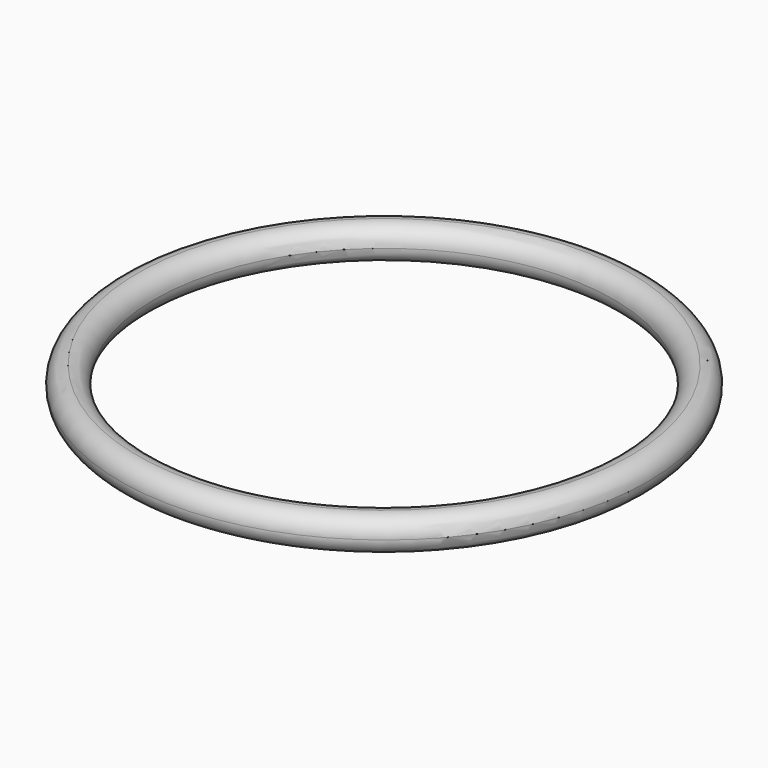
from build123d import *

# Parameters (mm, degrees)
F0_R     = 11.5
F0_R_2   = 10
F1_DEPTH = 1.5
F2_R     = 0.74999


# Not quite as in the source:
# - a fillet or chamfer is up to 0.001 mm smaller than in the source, because OpenCascade refuses the exact size


with BuildPart() as f1:
    # F0 (on Top) → F1 (new body)
    with BuildSketch(Plane.XY):
        Circle(F0_R)
        Circle(F0_R_2, mode=Mode.SUBTRACT)
    extrude(amount=F1_DEPTH)

    # F2 (radius 0.75 in the source; OpenCascade refuses exactly that, so slightly less here)
    f2_edges = [f1.edges().sort_by_distance(p)[0] for p in [
        (-10, 0, 1.5),
        (-11.5, 0, 1.5),
        (-11.5, 0, 0),
        (-10, 0, 0),
    ]]
    fillet(f2_edges, radius=F2_R)


solid = f1.part
